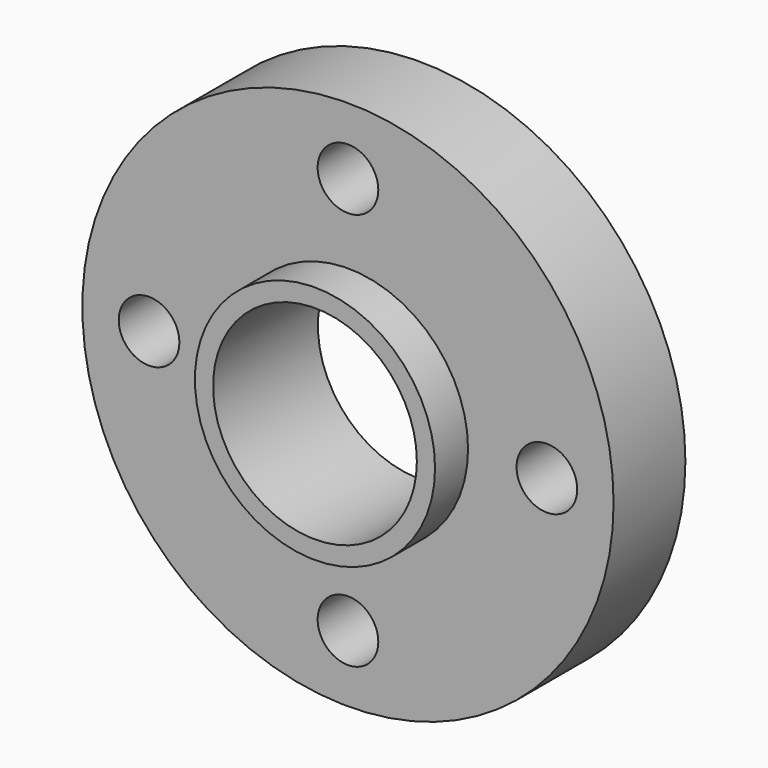
from build123d import *

# Parameters (mm, degrees)
F0_R     = 4.95
F0_R_2   = 4.2
F1_DEPTH = 5.4
F0_R_3   = 10.95
F0_R_4   = 1.25
F2_DEPTH = 3.7


# Not quite as in the source:
# - the program builds the solid bodies; features that only make, move or delete a surface that nothing else refers to are left out


with BuildPart() as f1:
    # F0 (on Front) → F1 (new body)
    with BuildSketch(Plane.XZ):
        Circle(F0_R)
        Circle(F0_R_2, mode=Mode.SUBTRACT)
    extrude(amount=F1_DEPTH)

    # F0 (on Front) → F2 (join)
    with BuildSketch(Plane.XZ):
        Circle(F0_R_3)
        with Locations((0, -8.2)):
            Circle(F0_R_4, mode=Mode.SUBTRACT)
        with Locations((-8.2, 0)):
            Circle(F0_R_4, mode=Mode.SUBTRACT)
        Circle(F0_R, mode=Mode.SUBTRACT)
        with Locations((8.2, 0)):
            Circle(F0_R_4, mode=Mode.SUBTRACT)
        with Locations((0, 8.2)):
            Circle(F0_R_4, mode=Mode.SUBTRACT)
    extrude(amount=F2_DEPTH)


solid = f1.part
